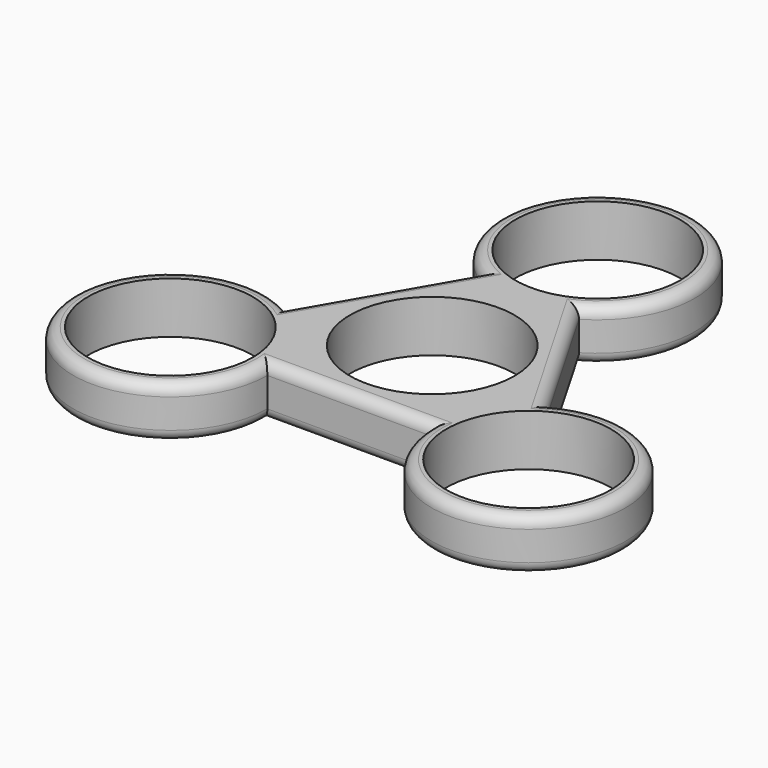
from build123d import *

# Parameters (mm, degrees)
F0_R     = 11.2
F1_DEPTH = 7
F2_R     = 1.5
F3_R     = 1.49999


# Not quite as in the source:
# - a fillet or chamfer is up to 0.001 mm smaller than in the source, because OpenCascade refuses the exact size


with BuildPart() as f1:
    # F0 (on Top) → F1 (new body)
    with BuildSketch(Plane.XY):
        with BuildLine():
            Line((17.7733109715, -2.6404023205), (6.6, 16.7123399709))
            ThreePointArc((6.6, 16.7123399709), (0, 41.3438753009), (-6.6, 16.7123399709))
            Line((-6.6, 16.7123399709), (-17.7733109715, -2.6404023205))
            ThreePointArc((-17.7733109715, -2.6404023205), (-35.8048463015, -20.6719376504), (-11.1733109715, -14.0719376504))
            Line((-11.1733109715, -14.0719376504), (11.1733109715, -14.0719376504))
            ThreePointArc((11.1733109715, -14.0719376504), (35.8048463015, -20.6719376504), (17.7733109715, -2.6404023205))
        make_face()
        with Locations((-24.3733109715, -14.0719376504)):
            Circle(F0_R, mode=Mode.SUBTRACT)
        with Locations((24.3733109715, -14.0719376504)):
            Circle(F0_R, mode=Mode.SUBTRACT)
        Circle(F0_R, mode=Mode.SUBTRACT)
        with Locations((0, 28.1438753009)):
            Circle(F0_R, mode=Mode.SUBTRACT)
    extrude(amount=F1_DEPTH)

    # F2
    f2_edges = [f1.edges().sort_by_distance(p)[0] for p in [
        (0, -14.071938, 7),
        (0, -14.071938, 0),
        (-35.804846, -20.671938, 7),
        (-12.186655, 7.035969, 7),
        (0, 41.343875, 7),
        (12.186655, 7.035969, 7),
        (35.804846, -20.671938, 7),
    ]]
    fillet(f2_edges, radius=F2_R)

    # F3 (radius 1.5 in the source; OpenCascade refuses exactly that, so slightly less here)
    f3_edges = [f1.edges().sort_by_distance(p)[0] for p in [
        (-35.804846, -20.671938, 0),
        (-12.186655, 7.035969, 0),
        (0, 41.343875, 0),
        (12.186655, 7.035969, 0),
        (35.804846, -20.671938, 0),
    ]]
    fillet(f3_edges, radius=F3_R)


solid = f1.part
